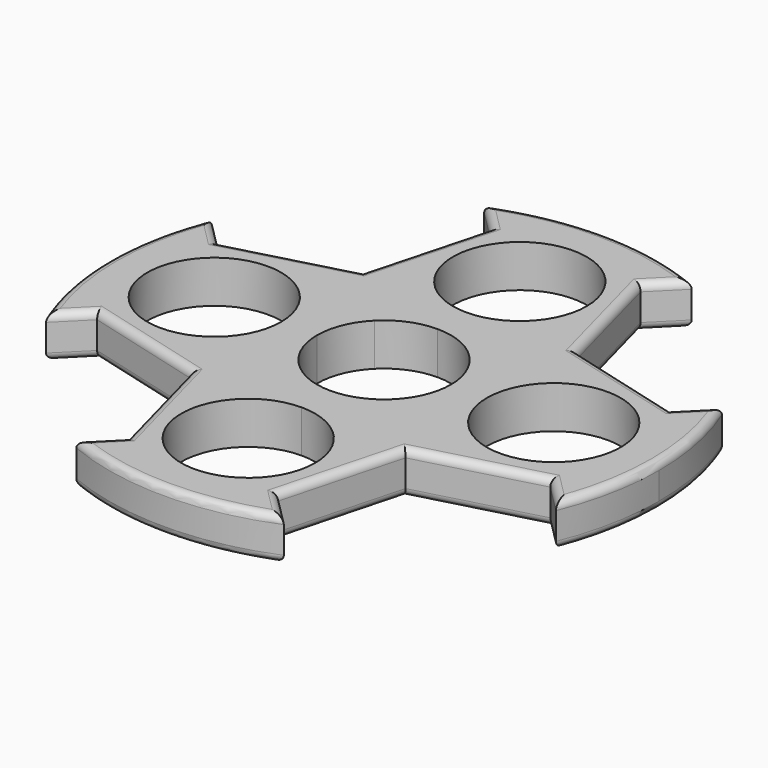
from build123d import *

# Parameters (mm, degrees)
F0_R          = 11.0109
F1_DEPTH      = 6.985
F2_T4_DEPTH   = 26.67
F2_T10_DEPTH  = 12.952299935
F2_T13_ANGLE  = 52.3145955419
F2_T17_DEPTH  = 12.952299935
F2_T22_DEPTH  = 26.67
F2_T28_DEPTH  = 26.67
F2_T34_DEPTH  = 26.67
F2_T40_DEPTH  = 12.952299935
F2_T45_DEPTH  = 12.952299935
F2_T50_DEPTH  = 26.67
F2_T54_ANGLE  = 52.3145955419
F2_T58_DEPTH  = 26.67
F2_T64_DEPTH  = 12.952299935
F2_T67_ANGLE  = 52.3145955419
F2_T71_DEPTH  = 12.952299935
F2_T76_DEPTH  = 26.67
F2_T82_DEPTH  = 26.67
F2_T88_DEPTH  = 12.952299935
F2_T93_DEPTH  = 12.952299935
F2_T96_ANGLE  = 52.3145955419
F2_T98_ANGLE  = 52.3145955419
F2_T102_DEPTH = 26.67
F2_T108_DEPTH = 26.67
F2_T114_DEPTH = 12.952299935
F2_T117_ANGLE = 52.3145955419
F2_T121_DEPTH = 26.67
F2_T127_DEPTH = 12.952299935
F2_T132_DEPTH = 26.67
F2_T138_DEPTH = 12.952299935
F2_T141_ANGLE = 52.3145955419
F2_T145_DEPTH = 12.952299935
F2_T150_DEPTH = 26.67
F2_T156_DEPTH = 26.67
F2_T162_DEPTH = 12.952299935
F2_T165_ANGLE = 52.3145955419
F2_T169_DEPTH = 26.67
F2_T175_DEPTH = 12.952299935
F2_T180_DEPTH = 26.67
F2_T186_DEPTH = 12.952299935
F2_T192_DEPTH = 12.952299935
F2_T196_DEPTH = 26.67
F2_T203_DEPTH = 26.67
F2_T207_DEPTH = 26.67
F2_T214_DEPTH = 26.67
F2_T218_DEPTH = 12.952299935
F2_T225_DEPTH = 26.67
F2_T229_DEPTH = 26.67
F2_T236_DEPTH = 12.952299935
F2_T240_DEPTH = 26.67
F2_T247_DEPTH = 26.67
F2_T251_DEPTH = 12.952299935
F2_T258_DEPTH = 12.952299935
F2_T262_DEPTH = 26.67
F2_T269_DEPTH = 26.67
F2_T273_DEPTH = 26.67
F2_T280_DEPTH = 26.67
F2_T284_DEPTH = 12.952299935
F2_T291_DEPTH = 12.952299935
F2_T295_DEPTH = 26.67
F2_T302_DEPTH = 26.67
F2_T306_DEPTH = 26.67
F2_T313_DEPTH = 26.67
F2_T317_DEPTH = 12.952299935
F2_T324_DEPTH = 26.67
F2_T328_DEPTH = 26.67
F2_T335_DEPTH = 26.67
F2_T339_DEPTH = 12.952299935
F2_T346_DEPTH = 12.952299935
F2_T350_DEPTH = 26.67
F2_T357_DEPTH = 26.67
F2_T361_DEPTH = 26.67
F2_T368_DEPTH = 26.67
F2_T372_DEPTH = 12.952299935
F2_T379_DEPTH = 12.952299935
F2_T383_DEPTH = 26.67
F2_T390_DEPTH = 26.67
F2_T394_DEPTH = 26.67
F2_T401_DEPTH = 26.67
F2_T405_DEPTH = 12.952299935
F2_T412_DEPTH = 12.952299935
F2_T416_DEPTH = 26.67
F2_T423_DEPTH = 26.67
F2_T427_DEPTH = 26.67
F2_T434_DEPTH = 26.67
F2_T438_DEPTH = 12.952299935


# Not quite as in the source:
# - a fillet or chamfer that OpenCascade refuses, or shapes differently, is made with other operations: its cross-section is extruded or revolved along the edge and cut away or added


with BuildPart() as f1:
    # F0 (on Top) → F1 (new body)
    with BuildSketch(Plane.XY):
        with BuildLine():
            ThreePointArc((7.785882057, 7.785882057), (10.1727451445, 4.2136890054), (11.0109, 0))
            ThreePointArc((11.0109, 0), (10.1727451445, -4.2136890054), (7.785882057, -7.785882057))
            Line((7.785882057, -7.785882057), (17.6641637901, -17.6641637901))
            Line((17.6641637901, -17.6641637901), (37.2917765803, -12.4049607937))
            Line((37.2917765803, -12.4049607937), (41.9603076358, -17.0734918491))
            ThreePointArc((41.9603076358, -17.0734918491), (44.4579084134, -8.698616), (45.3009, 0))
            ThreePointArc((45.3009, 0), (44.4579084134, 8.698616), (41.9603076358, 17.0734918491))
            Line((41.9603076358, 17.0734918491), (37.2917765803, 12.4049607937))
            Line((37.2917765803, 12.4049607937), (17.6641637901, 17.6641637901))
            Line((17.6641637901, 17.6641637901), (7.785882057, 7.785882057))
        make_face()
        with BuildLine():
            ThreePointArc((38.9509, 0), (27.94, -11.0109), (16.9291, 0))
            ThreePointArc((16.9291, 0), (27.94, 11.0109), (38.9509, 0))
        make_face(mode=Mode.SUBTRACT)
        with BuildLine():
            ThreePointArc((0, 11.0109), (4.2136890054, 10.1727451445), (7.785882057, 7.785882057))
            Line((7.785882057, 7.785882057), (17.6641637901, 17.6641637901))
            Line((17.6641637901, 17.6641637901), (12.4049607937, 37.2917765803))
            Line((12.4049607937, 37.2917765803), (17.0734918491, 41.9603076358))
            ThreePointArc((17.0734918491, 41.9603076358), (0, 45.3009), (-17.0734918491, 41.9603076358))
            Line((-17.0734918491, 41.9603076358), (-12.4049607937, 37.2917765803))
            Line((-12.4049607937, 37.2917765803), (-17.6641637901, 17.6641637901))
            Line((-17.6641637901, 17.6641637901), (-7.785882057, 7.785882057))
            ThreePointArc((-7.785882057, 7.785882057), (-4.2136890054, 10.1727451445), (0, 11.0109))
        make_face()
        with BuildLine():
            ThreePointArc((11.0109, 27.94), (7.785882057, 20.154117943), (0, 16.9291))
            ThreePointArc((0, 16.9291), (-7.785882057, 35.725882057), (11.0109, 27.94))
        make_face(mode=Mode.SUBTRACT)
        with BuildLine():
            ThreePointArc((-7.785882057, -7.785882057), (-10.1727451445, -4.2136890054), (-11.0109, 0))
            ThreePointArc((-11.0109, 0), (-10.1727451445, 4.2136890054), (-7.785882057, 7.785882057))
            Line((-7.785882057, 7.785882057), (-17.6641637901, 17.6641637901))
            Line((-17.6641637901, 17.6641637901), (-37.2917765803, 12.4049607937))
            Line((-37.2917765803, 12.4049607937), (-41.9603076358, 17.0734918491))
            ThreePointArc((-41.9603076358, 17.0734918491), (-45.3009, 0), (-41.9603076358, -17.0734918491))
            Line((-41.9603076358, -17.0734918491), (-37.2917765803, -12.4049607937))
            Line((-37.2917765803, -12.4049607937), (-17.6641637901, -17.6641637901))
            Line((-17.6641637901, -17.6641637901), (-7.785882057, -7.785882057))
        make_face()
        with Locations((-27.94, 0)):
            Circle(F0_R, mode=Mode.SUBTRACT)
        with BuildLine():
            Line((17.6641637901, -17.6641637901), (7.785882057, -7.785882057))
            ThreePointArc((7.785882057, -7.785882057), (4.2136890054, -10.1727451445), (0, -11.0109))
            ThreePointArc((0, -11.0109), (-4.2136890054, -10.1727451445), (-7.785882057, -7.785882057))
            Line((-7.785882057, -7.785882057), (-17.6641637901, -17.6641637901))
            Line((-17.6641637901, -17.6641637901), (-12.4049607937, -37.2917765803))
            Line((-12.4049607937, -37.2917765803), (-17.0734918491, -41.9603076358))
            ThreePointArc((-17.0734918491, -41.9603076358), (0, -45.3009), (17.0734918491, -41.9603076358))
            Line((17.0734918491, -41.9603076358), (12.4049607937, -37.2917765803))
            Line((12.4049607937, -37.2917765803), (17.6641637901, -17.6641637901))
        make_face()
        with BuildLine():
            ThreePointArc((11.0109, -27.94), (-7.785882057, -35.725882057), (0, -16.9291))
            ThreePointArc((0, -16.9291), (7.785882057, -20.154117943), (11.0109, -27.94))
        make_face(mode=Mode.SUBTRACT)
    extrude(amount=F1_DEPTH)

    # F2: fillet of radius 1.27 on 39 edges, made by hand


with BuildPart() as f2_tool2:
    # F2_s3 → F2_t4 (new body)
    with BuildSketch(Plane(origin=(9.3137198066, 34.7592755256, 0), x_dir=(0, 0, 1), z_dir=(-0.2588190451, -0.9659258263, 0))):
        with BuildLine():
            ThreePointArc((5.715, 21.6340940094), (6.6130256121, 21.2621196215), (6.985, 20.3640940094))
            Line((6.985, 20.3640940094), (6.985, 21.6340940094))
            Line((6.985, 21.6340940094), (5.715, 21.6340940094))
        make_face()
    extrude(amount=F2_T4_DEPTH)

    split(bisect_by=Plane(origin=(12.4434078933, 12.4434078933, 0), x_dir=(0, 0, 1), z_dir=(-0.7071067812, -0.7071067812, 0)), keep=Keep.TOP)

    split(bisect_by=Plane(origin=(-5.5993155532, 20.896930132, 0), x_dir=(0, 0, 1), z_dir=(-0.2588190451, 0.9659258263, 0)), keep=Keep.TOP)


with BuildPart() as f1_1:
    add(f1.part)

    # F2_t1: cut F2_tool2
    add(f2_tool2.part, mode=Mode.SUBTRACT)


with BuildPart() as f2_tool8:
    # F2_s9 → F2_t10 (new body)
    with BuildSketch(Plane(origin=(-31.7619637727, 31.7619637727, 0), x_dir=(0, 0, 1), z_dir=(0.7071067812, -0.7071067812, 0))):
        with BuildLine():
            ThreePointArc((5.715, -17.5976362049), (6.6130256121, -17.9696105928), (6.985, -18.8676362049))
            Line((6.985, -18.8676362049), (6.985, -17.5976362049))
            Line((6.985, -17.5976362049), (5.715, -17.5976362049))
        make_face()
    extrude(amount=F2_T10_DEPTH)

    split(bisect_by=Plane(origin=(-20.896930132, 5.5993155532, 0), x_dir=(0, 0, 1), z_dir=(-0.9659258263, 0.2588190451, 0)), keep=Keep.TOP)


with BuildPart() as f1_2:
    add(f1_1.part)

    # F2_t7: cut F2_tool8
    add(f2_tool8.part, mode=Mode.SUBTRACT)

    # F2_s12 → F2_t13 (revolve, cut)
    with BuildSketch(Plane(origin=(0, 0, 0), x_dir=(0, 0, 1), z_dir=(0.8975871723, -0.4408370085, 0))):
        with BuildLine():
            ThreePointArc((5.715, -45.3009), (6.6130256121, -44.9289256121), (6.985, -44.0309))
            Line((6.985, -44.0309), (6.985, -45.3009))
            Line((6.985, -45.3009), (5.715, -45.3009))
        make_face()
    revolve(axis=Axis((0, 0, 6.985), (0, 0, 1)), revolution_arc=F2_T13_ANGLE, mode=Mode.SUBTRACT)


with BuildPart() as f2_tool15:
    # F2_s16 → F2_t17 (new body)
    with BuildSketch(Plane(origin=(22.6033046567, 22.6033046567, 0), x_dir=(0, 0, 1), z_dir=(0.7071067812, 0.7071067812, 0))):
        with BuildLine():
            ThreePointArc((5.715, -17.5976362049), (6.6130256121, -17.9696105928), (6.985, -18.8676362049))
            Line((6.985, -18.8676362049), (6.985, -17.5976362049))
            Line((6.985, -17.5976362049), (5.715, -17.5976362049))
        make_face()
    extrude(amount=F2_T17_DEPTH)

    split(bisect_by=Plane(origin=(20.896930132, 5.5993155532, 0), x_dir=(0, 0, 1), z_dir=(0.9659258263, 0.2588190451, 0)), keep=Keep.TOP)


with BuildPart() as f1_3:
    add(f1_2.part)

    # F2_t14: cut F2_tool15
    add(f2_tool15.part, mode=Mode.SUBTRACT)


with BuildPart() as f2_tool20:
    # F2_s21 → F2_t22 (new body)
    with BuildSketch(Plane(origin=(-2.4110158737, 8.9980337385, 0), x_dir=(0, 0, 1), z_dir=(-0.2588190451, 0.9659258263, 0))):
        with BuildLine():
            ThreePointArc((5.715, 21.6340940094), (6.6130256121, 21.2621196215), (6.985, 20.3640940094))
            Line((6.985, 20.3640940094), (6.985, 21.6340940094))
            Line((6.985, 21.6340940094), (5.715, 21.6340940094))
        make_face()
    extrude(amount=F2_T22_DEPTH)

    split(bisect_by=Plane(origin=(5.5993155532, 20.896930132, 0), x_dir=(0, 0, 1), z_dir=(0.2588190451, 0.9659258263, 0)), keep=Keep.TOP)

    split(bisect_by=Plane(origin=(-12.4434078933, 12.4434078933, 0), x_dir=(0, 0, 1), z_dir=(0.7071067812, -0.7071067812, 0)), keep=Keep.TOP)


with BuildPart() as f1_4:
    add(f1_3.part)

    # F2_t19: cut F2_tool20
    add(f2_tool20.part, mode=Mode.SUBTRACT)


with BuildPart() as f2_tool26:
    # F2_s27 → F2_t28 (new body)
    with BuildSketch(Plane(origin=(34.7592755256, -9.3137198066, 0), x_dir=(0, 0, 1), z_dir=(-0.9659258263, 0.2588190451, 0))):
        with BuildLine():
            ThreePointArc((5.715, 21.6340940094), (6.6130256121, 21.2621196215), (6.985, 20.3640940094))
            Line((6.985, 20.3640940094), (6.985, 21.6340940094))
            Line((6.985, 21.6340940094), (5.715, 21.6340940094))
        make_face()
    extrude(amount=F2_T28_DEPTH)

    split(bisect_by=Plane(origin=(12.4434078933, -12.4434078933, 0), x_dir=(0, 0, 1), z_dir=(-0.7071067812, 0.7071067812, 0)), keep=Keep.TOP)

    split(bisect_by=Plane(origin=(20.896930132, 5.5993155532, 0), x_dir=(0, 0, 1), z_dir=(0.9659258263, 0.2588190451, 0)), keep=Keep.TOP)


with BuildPart() as f1_5:
    add(f1_4.part)

    # F2_t25: cut F2_tool26
    add(f2_tool26.part, mode=Mode.SUBTRACT)


with BuildPart() as f2_tool32:
    # F2_s33 → F2_t34 (new body)
    with BuildSketch(Plane(origin=(-8.9980337385, -2.4110158737, 0), x_dir=(0, 0, 1), z_dir=(-0.9659258263, -0.2588190451, 0))):
        with BuildLine():
            ThreePointArc((5.715, 21.6340940094), (6.6130256121, 21.2621196215), (6.985, 20.3640940094))
            Line((6.985, 20.3640940094), (6.985, 21.6340940094))
            Line((6.985, 21.6340940094), (5.715, 21.6340940094))
        make_face()
    extrude(amount=F2_T34_DEPTH)

    split(bisect_by=Plane(origin=(-20.896930132, 5.5993155532, 0), x_dir=(0, 0, 1), z_dir=(-0.9659258263, 0.2588190451, 0)), keep=Keep.TOP)

    split(bisect_by=Plane(origin=(-12.4434078933, -12.4434078933, 0), x_dir=(0, 0, 1), z_dir=(0.7071067812, 0.7071067812, 0)), keep=Keep.TOP)


with BuildPart() as f1_6:
    add(f1_5.part)

    # F2_t31: cut F2_tool32
    add(f2_tool32.part, mode=Mode.SUBTRACT)


with BuildPart() as f2_tool38:
    # F2_s39 → F2_t40 (new body)
    with BuildSketch(Plane(origin=(-22.6033046567, 22.6033046567, 0), x_dir=(0, 0, 1), z_dir=(-0.7071067812, 0.7071067812, 0))):
        with BuildLine():
            ThreePointArc((5.715, -17.5976362049), (6.6130256121, -17.9696105928), (6.985, -18.8676362049))
            Line((6.985, -18.8676362049), (6.985, -17.5976362049))
            Line((6.985, -17.5976362049), (5.715, -17.5976362049))
        make_face()
    extrude(amount=F2_T40_DEPTH)

    split(bisect_by=Plane(origin=(-5.5993155532, 20.896930132, 0), x_dir=(0, 0, 1), z_dir=(-0.2588190451, 0.9659258263, 0)), keep=Keep.TOP)


with BuildPart() as f1_7:
    add(f1_6.part)

    # F2_t37: cut F2_tool38
    add(f2_tool38.part, mode=Mode.SUBTRACT)


with BuildPart() as f2_tool43:
    # F2_s44 → F2_t45 (new body)
    with BuildSketch(Plane(origin=(-31.7619637727, -31.7619637727, 0), x_dir=(0, 0, 1), z_dir=(0.7071067812, 0.7071067812, 0))):
        with BuildLine():
            ThreePointArc((5.715, -17.5976362049), (6.6130256121, -17.9696105928), (6.985, -18.8676362049))
            Line((6.985, -18.8676362049), (6.985, -17.5976362049))
            Line((6.985, -17.5976362049), (5.715, -17.5976362049))
        make_face()
    extrude(amount=F2_T45_DEPTH)

    split(bisect_by=Plane(origin=(-5.5993155532, -20.896930132, 0), x_dir=(0, 0, 1), z_dir=(-0.2588190451, -0.9659258263, 0)), keep=Keep.TOP)


with BuildPart() as f1_8:
    add(f1_7.part)

    # F2_t42: cut F2_tool43
    add(f2_tool43.part, mode=Mode.SUBTRACT)


with BuildPart() as f2_tool48:
    # F2_s49 → F2_t50 (new body)
    with BuildSketch(Plane(origin=(-34.7592755256, 9.3137198066, 0), x_dir=(0, 0, 1), z_dir=(0.9659258263, -0.2588190451, 0))):
        with BuildLine():
            ThreePointArc((5.715, 21.6340940094), (6.6130256121, 21.2621196215), (6.985, 20.3640940094))
            Line((6.985, 20.3640940094), (6.985, 21.6340940094))
            Line((6.985, 21.6340940094), (5.715, 21.6340940094))
        make_face()
    extrude(amount=F2_T50_DEPTH)

    split(bisect_by=Plane(origin=(-12.4434078933, 12.4434078933, 0), x_dir=(0, 0, 1), z_dir=(0.7071067812, -0.7071067812, 0)), keep=Keep.TOP)

    split(bisect_by=Plane(origin=(-20.896930132, -5.5993155532, 0), x_dir=(0, 0, 1), z_dir=(-0.9659258263, -0.2588190451, 0)), keep=Keep.TOP)


with BuildPart() as f1_9:
    add(f1_8.part)

    # F2_t47: cut F2_tool48
    add(f2_tool48.part, mode=Mode.SUBTRACT)

    # F2_s53 → F2_t54 (revolve, cut)
    with BuildSketch(Plane(origin=(0, 0, 0), x_dir=(0, 0, 1), z_dir=(0.4408370085, 0.8975871723, 0))):
        with BuildLine():
            ThreePointArc((5.715, -45.3009), (6.6130256121, -44.9289256121), (6.985, -44.0309))
            Line((6.985, -44.0309), (6.985, -45.3009))
            Line((6.985, -45.3009), (5.715, -45.3009))
        make_face()
    revolve(axis=Axis((0, 0, 6.985), (0, 0, 1)), revolution_arc=F2_T54_ANGLE, mode=Mode.SUBTRACT)


with BuildPart() as f2_tool56:
    # F2_s57 → F2_t58 (new body)
    with BuildSketch(Plane(origin=(2.4110158737, -8.9980337385, 0), x_dir=(0, 0, 1), z_dir=(0.2588190451, -0.9659258263, 0))):
        with BuildLine():
            ThreePointArc((5.715, 21.6340940094), (6.6130256121, 21.2621196215), (6.985, 20.3640940094))
            Line((6.985, 20.3640940094), (6.985, 21.6340940094))
            Line((6.985, 21.6340940094), (5.715, 21.6340940094))
        make_face()
    extrude(amount=F2_T58_DEPTH)

    split(bisect_by=Plane(origin=(-5.5993155532, -20.896930132, 0), x_dir=(0, 0, 1), z_dir=(-0.2588190451, -0.9659258263, 0)), keep=Keep.TOP)

    split(bisect_by=Plane(origin=(12.4434078933, -12.4434078933, 0), x_dir=(0, 0, 1), z_dir=(-0.7071067812, 0.7071067812, 0)), keep=Keep.TOP)


with BuildPart() as f1_10:
    add(f1_9.part)

    # F2_t55: cut F2_tool56
    add(f2_tool56.part, mode=Mode.SUBTRACT)


with BuildPart() as f2_tool62:
    # F2_s63 → F2_t64 (new body)
    with BuildSketch(Plane(origin=(-22.6033046567, -22.6033046567, 0), x_dir=(0, 0, 1), z_dir=(-0.7071067812, -0.7071067812, 0))):
        with BuildLine():
            ThreePointArc((5.715, -17.5976362049), (6.6130256121, -17.9696105928), (6.985, -18.8676362049))
            Line((6.985, -18.8676362049), (6.985, -17.5976362049))
            Line((6.985, -17.5976362049), (5.715, -17.5976362049))
        make_face()
    extrude(amount=F2_T64_DEPTH)

    split(bisect_by=Plane(origin=(-20.896930132, -5.5993155532, 0), x_dir=(0, 0, 1), z_dir=(-0.9659258263, -0.2588190451, 0)), keep=Keep.TOP)


with BuildPart() as f1_11:
    add(f1_10.part)

    # F2_t61: cut F2_tool62
    add(f2_tool62.part, mode=Mode.SUBTRACT)

    # F2_s66 → F2_t67 (revolve, cut)
    with BuildSketch(Plane(origin=(0, 0, 0), x_dir=(0, 0, 1), z_dir=(-0.8975871723, 0.4408370085, 0))):
        with BuildLine():
            ThreePointArc((5.715, -45.3009), (6.6130256121, -44.9289256121), (6.985, -44.0309))
            Line((6.985, -44.0309), (6.985, -45.3009))
            Line((6.985, -45.3009), (5.715, -45.3009))
        make_face()
    revolve(axis=Axis((0, 0, 6.985), (0, 0, 1)), revolution_arc=F2_T67_ANGLE, mode=Mode.SUBTRACT)


with BuildPart() as f2_tool69:
    # F2_s70 → F2_t71 (new body)
    with BuildSketch(Plane(origin=(31.7619637727, -31.7619637727, 0), x_dir=(0, 0, 1), z_dir=(-0.7071067812, 0.7071067812, 0))):
        with BuildLine():
            ThreePointArc((5.715, -17.5976362049), (6.6130256121, -17.9696105928), (6.985, -18.8676362049))
            Line((6.985, -18.8676362049), (6.985, -17.5976362049))
            Line((6.985, -17.5976362049), (5.715, -17.5976362049))
        make_face()
    extrude(amount=F2_T71_DEPTH)

    split(bisect_by=Plane(origin=(20.896930132, -5.5993155532, 0), x_dir=(0, 0, 1), z_dir=(0.9659258263, -0.2588190451, 0)), keep=Keep.TOP)


with BuildPart() as f1_12:
    add(f1_11.part)

    # F2_t68: cut F2_tool69
    add(f2_tool69.part, mode=Mode.SUBTRACT)


with BuildPart() as f2_tool74:
    # F2_s75 → F2_t76 (new body)
    with BuildSketch(Plane(origin=(-9.3137198066, -34.7592755256, 0), x_dir=(0, 0, 1), z_dir=(0.2588190451, 0.9659258263, 0))):
        with BuildLine():
            ThreePointArc((5.715, 21.6340940094), (6.6130256121, 21.2621196215), (6.985, 20.3640940094))
            Line((6.985, 20.3640940094), (6.985, 21.6340940094))
            Line((6.985, 21.6340940094), (5.715, 21.6340940094))
        make_face()
    extrude(amount=F2_T76_DEPTH)

    split(bisect_by=Plane(origin=(-12.4434078933, -12.4434078933, 0), x_dir=(0, 0, 1), z_dir=(0.7071067812, 0.7071067812, 0)), keep=Keep.TOP)

    split(bisect_by=Plane(origin=(5.5993155532, -20.896930132, 0), x_dir=(0, 0, 1), z_dir=(0.2588190451, -0.9659258263, 0)), keep=Keep.TOP)


with BuildPart() as f1_13:
    add(f1_12.part)

    # F2_t73: cut F2_tool74
    add(f2_tool74.part, mode=Mode.SUBTRACT)


with BuildPart() as f2_tool80:
    # F2_s81 → F2_t82 (new body)
    with BuildSketch(Plane(origin=(8.9980337385, 2.4110158737, 0), x_dir=(0, 0, 1), z_dir=(0.9659258263, 0.2588190451, 0))):
        with BuildLine():
            ThreePointArc((5.715, 21.6340940094), (6.6130256121, 21.2621196215), (6.985, 20.3640940094))
            Line((6.985, 20.3640940094), (6.985, 21.6340940094))
            Line((6.985, 21.6340940094), (5.715, 21.6340940094))
        make_face()
    extrude(amount=F2_T82_DEPTH)

    split(bisect_by=Plane(origin=(20.896930132, -5.5993155532, 0), x_dir=(0, 0, 1), z_dir=(0.9659258263, -0.2588190451, 0)), keep=Keep.TOP)

    split(bisect_by=Plane(origin=(12.4434078933, 12.4434078933, 0), x_dir=(0, 0, 1), z_dir=(-0.7071067812, -0.7071067812, 0)), keep=Keep.TOP)


with BuildPart() as f1_14:
    add(f1_13.part)

    # F2_t79: cut F2_tool80
    add(f2_tool80.part, mode=Mode.SUBTRACT)


with BuildPart() as f2_tool86:
    # F2_s87 → F2_t88 (new body)
    with BuildSketch(Plane(origin=(22.6033046567, -22.6033046567, 0), x_dir=(0, 0, 1), z_dir=(0.7071067812, -0.7071067812, 0))):
        with BuildLine():
            ThreePointArc((5.715, -17.5976362049), (6.6130256121, -17.9696105928), (6.985, -18.8676362049))
            Line((6.985, -18.8676362049), (6.985, -17.5976362049))
            Line((6.985, -17.5976362049), (5.715, -17.5976362049))
        make_face()
    extrude(amount=F2_T88_DEPTH)

    split(bisect_by=Plane(origin=(5.5993155532, -20.896930132, 0), x_dir=(0, 0, 1), z_dir=(0.2588190451, -0.9659258263, 0)), keep=Keep.TOP)


with BuildPart() as f1_15:
    add(f1_14.part)

    # F2_t85: cut F2_tool86
    add(f2_tool86.part, mode=Mode.SUBTRACT)


with BuildPart() as f2_tool91:
    # F2_s92 → F2_t93 (new body)
    with BuildSketch(Plane(origin=(31.7619637727, 31.7619637727, 0), x_dir=(0, 0, 1), z_dir=(-0.7071067812, -0.7071067812, 0))):
        with BuildLine():
            ThreePointArc((5.715, -17.5976362049), (6.6130256121, -17.9696105928), (6.985, -18.8676362049))
            Line((6.985, -18.8676362049), (6.985, -17.5976362049))
            Line((6.985, -17.5976362049), (5.715, -17.5976362049))
        make_face()
    extrude(amount=F2_T93_DEPTH)

    split(bisect_by=Plane(origin=(5.5993155532, 20.896930132, 0), x_dir=(0, 0, 1), z_dir=(0.2588190451, 0.9659258263, 0)), keep=Keep.TOP)


with BuildPart() as f1_16:
    add(f1_15.part)

    # F2_t90: cut F2_tool91
    add(f2_tool91.part, mode=Mode.SUBTRACT)

    # F2_s95 → F2_t96 (revolve, cut)
    with BuildSketch(Plane(origin=(0, 0, 0), x_dir=(0, 0, 1), z_dir=(-0.4408370085, -0.8975871723, 0))):
        with BuildLine():
            ThreePointArc((5.715, -45.3009), (6.6130256121, -44.9289256121), (6.985, -44.0309))
            Line((6.985, -44.0309), (6.985, -45.3009))
            Line((6.985, -45.3009), (5.715, -45.3009))
        make_face()
    revolve(axis=Axis((0, 0, 6.985), (0, 0, 1)), revolution_arc=F2_T96_ANGLE, mode=Mode.SUBTRACT)

    # F2_s97 → F2_t98 (revolve, cut)
    with BuildSketch(Plane(origin=(0, 0, 0), x_dir=(0, 0, 1), z_dir=(0.8975871723, -0.4408370085, 0))):
        with BuildLine():
            ThreePointArc((1.27, -45.3009), (0.3719743879, -44.9289256121), (0, -44.0309))
            Line((0, -44.0309), (0, -45.3009))
            Line((0, -45.3009), (1.27, -45.3009))
        make_face()
    revolve(axis=Axis((0, 0, 0), (0, 0, 1)), revolution_arc=F2_T98_ANGLE, mode=Mode.SUBTRACT)


with BuildPart() as f2_tool100:
    # F2_s101 → F2_t102 (new body)
    with BuildSketch(Plane(origin=(9.3137198066, 34.7592755256, 0), x_dir=(0, 0, 1), z_dir=(-0.2588190451, -0.9659258263, 0))):
        with BuildLine():
            ThreePointArc((1.27, 21.6340940094), (0.3719743879, 21.2621196215), (0, 20.3640940094))
            Line((0, 20.3640940094), (0, 21.6340940094))
            Line((0, 21.6340940094), (1.27, 21.6340940094))
        make_face()
    extrude(amount=F2_T102_DEPTH)

    split(bisect_by=Plane(origin=(12.4434078933, 12.4434078933, 0), x_dir=(0, 0, 1), z_dir=(-0.7071067812, -0.7071067812, 0)), keep=Keep.TOP)

    split(bisect_by=Plane(origin=(-5.5993155532, 20.896930132, 0), x_dir=(0, 0, 1), z_dir=(-0.2588190451, 0.9659258263, 0)), keep=Keep.TOP)


with BuildPart() as f1_17:
    add(f1_16.part)

    # F2_t99: cut F2_tool100
    add(f2_tool100.part, mode=Mode.SUBTRACT)


with BuildPart() as f2_tool106:
    # F2_s107 → F2_t108 (new body)
    with BuildSketch(Plane(origin=(-8.9980337385, -2.4110158737, 0), x_dir=(0, 0, 1), z_dir=(-0.9659258263, -0.2588190451, 0))):
        with BuildLine():
            ThreePointArc((1.27, 21.6340940094), (0.3719743879, 21.2621196215), (0, 20.3640940094))
            Line((0, 20.3640940094), (0, 21.6340940094))
            Line((0, 21.6340940094), (1.27, 21.6340940094))
        make_face()
    extrude(amount=F2_T108_DEPTH)

    split(bisect_by=Plane(origin=(-20.896930132, 5.5993155532, 0), x_dir=(0, 0, 1), z_dir=(-0.9659258263, 0.2588190451, 0)), keep=Keep.TOP)

    split(bisect_by=Plane(origin=(-12.4434078933, -12.4434078933, 0), x_dir=(0, 0, 1), z_dir=(0.7071067812, 0.7071067812, 0)), keep=Keep.TOP)


with BuildPart() as f1_18:
    add(f1_17.part)

    # F2_t105: cut F2_tool106
    add(f2_tool106.part, mode=Mode.SUBTRACT)


with BuildPart() as f2_tool112:
    # F2_s113 → F2_t114 (new body)
    with BuildSketch(Plane(origin=(-22.6033046567, 22.6033046567, 0), x_dir=(0, 0, 1), z_dir=(-0.7071067812, 0.7071067812, 0))):
        with BuildLine():
            ThreePointArc((1.27, -17.5976362049), (0.3719743879, -17.9696105928), (0, -18.8676362049))
            Line((0, -18.8676362049), (0, -17.5976362049))
            Line((0, -17.5976362049), (1.27, -17.5976362049))
        make_face()
    extrude(amount=F2_T114_DEPTH)

    split(bisect_by=Plane(origin=(-5.5993155532, 20.896930132, 0), x_dir=(0, 0, 1), z_dir=(-0.2588190451, 0.9659258263, 0)), keep=Keep.TOP)


with BuildPart() as f1_19:
    add(f1_18.part)

    # F2_t111: cut F2_tool112
    add(f2_tool112.part, mode=Mode.SUBTRACT)

    # F2_s116 → F2_t117 (revolve, cut)
    with BuildSketch(Plane(origin=(0, 0, 0), x_dir=(0, 0, 1), z_dir=(0.4408370085, 0.8975871723, 0))):
        with BuildLine():
            ThreePointArc((1.27, -45.3009), (0.3719743879, -44.9289256121), (0, -44.0309))
            Line((0, -44.0309), (0, -45.3009))
            Line((0, -45.3009), (1.27, -45.3009))
        make_face()
    revolve(axis=Axis((0, 0, 0), (0, 0, 1)), revolution_arc=F2_T117_ANGLE, mode=Mode.SUBTRACT)


with BuildPart() as f2_tool119:
    # F2_s120 → F2_t121 (new body)
    with BuildSketch(Plane(origin=(-34.7592755256, 9.3137198066, 0), x_dir=(0, 0, 1), z_dir=(0.9659258263, -0.2588190451, 0))):
        with BuildLine():
            ThreePointArc((1.27, 21.6340940094), (0.3719743879, 21.2621196215), (0, 20.3640940094))
            Line((0, 20.3640940094), (0, 21.6340940094))
            Line((0, 21.6340940094), (1.27, 21.6340940094))
        make_face()
    extrude(amount=F2_T121_DEPTH)

    split(bisect_by=Plane(origin=(-12.4434078933, 12.4434078933, 0), x_dir=(0, 0, 1), z_dir=(0.7071067812, -0.7071067812, 0)), keep=Keep.TOP)

    split(bisect_by=Plane(origin=(-20.896930132, -5.5993155532, 0), x_dir=(0, 0, 1), z_dir=(-0.9659258263, -0.2588190451, 0)), keep=Keep.TOP)


with BuildPart() as f1_20:
    add(f1_19.part)

    # F2_t118: cut F2_tool119
    add(f2_tool119.part, mode=Mode.SUBTRACT)


with BuildPart() as f2_tool125:
    # F2_s126 → F2_t127 (new body)
    with BuildSketch(Plane(origin=(-31.7619637727, -31.7619637727, 0), x_dir=(0, 0, 1), z_dir=(0.7071067812, 0.7071067812, 0))):
        with BuildLine():
            ThreePointArc((1.27, -17.5976362049), (0.3719743879, -17.9696105928), (0, -18.8676362049))
            Line((0, -18.8676362049), (0, -17.5976362049))
            Line((0, -17.5976362049), (1.27, -17.5976362049))
        make_face()
    extrude(amount=F2_T127_DEPTH)

    split(bisect_by=Plane(origin=(-5.5993155532, -20.896930132, 0), x_dir=(0, 0, 1), z_dir=(-0.2588190451, -0.9659258263, 0)), keep=Keep.TOP)


with BuildPart() as f1_21:
    add(f1_20.part)

    # F2_t124: cut F2_tool125
    add(f2_tool125.part, mode=Mode.SUBTRACT)


with BuildPart() as f2_tool130:
    # F2_s131 → F2_t132 (new body)
    with BuildSketch(Plane(origin=(2.4110158737, -8.9980337385, 0), x_dir=(0, 0, 1), z_dir=(0.2588190451, -0.9659258263, 0))):
        with BuildLine():
            ThreePointArc((1.27, 21.6340940094), (0.3719743879, 21.2621196215), (0, 20.3640940094))
            Line((0, 20.3640940094), (0, 21.6340940094))
            Line((0, 21.6340940094), (1.27, 21.6340940094))
        make_face()
    extrude(amount=F2_T132_DEPTH)

    split(bisect_by=Plane(origin=(-5.5993155532, -20.896930132, 0), x_dir=(0, 0, 1), z_dir=(-0.2588190451, -0.9659258263, 0)), keep=Keep.TOP)

    split(bisect_by=Plane(origin=(12.4434078933, -12.4434078933, 0), x_dir=(0, 0, 1), z_dir=(-0.7071067812, 0.7071067812, 0)), keep=Keep.TOP)


with BuildPart() as f1_22:
    add(f1_21.part)

    # F2_t129: cut F2_tool130
    add(f2_tool130.part, mode=Mode.SUBTRACT)


with BuildPart() as f2_tool136:
    # F2_s137 → F2_t138 (new body)
    with BuildSketch(Plane(origin=(-22.6033046567, -22.6033046567, 0), x_dir=(0, 0, 1), z_dir=(-0.7071067812, -0.7071067812, 0))):
        with BuildLine():
            ThreePointArc((1.27, -17.5976362049), (0.3719743879, -17.9696105928), (0, -18.8676362049))
            Line((0, -18.8676362049), (0, -17.5976362049))
            Line((0, -17.5976362049), (1.27, -17.5976362049))
        make_face()
    extrude(amount=F2_T138_DEPTH)

    split(bisect_by=Plane(origin=(-20.896930132, -5.5993155532, 0), x_dir=(0, 0, 1), z_dir=(-0.9659258263, -0.2588190451, 0)), keep=Keep.TOP)


with BuildPart() as f1_23:
    add(f1_22.part)

    # F2_t135: cut F2_tool136
    add(f2_tool136.part, mode=Mode.SUBTRACT)

    # F2_s140 → F2_t141 (revolve, cut)
    with BuildSketch(Plane(origin=(0, 0, 0), x_dir=(0, 0, 1), z_dir=(-0.8975871723, 0.4408370085, 0))):
        with BuildLine():
            ThreePointArc((1.27, -45.3009), (0.3719743879, -44.9289256121), (0, -44.0309))
            Line((0, -44.0309), (0, -45.3009))
            Line((0, -45.3009), (1.27, -45.3009))
        make_face()
    revolve(axis=Axis((0, 0, 0), (0, 0, 1)), revolution_arc=F2_T141_ANGLE, mode=Mode.SUBTRACT)


with BuildPart() as f2_tool143:
    # F2_s144 → F2_t145 (new body)
    with BuildSketch(Plane(origin=(31.7619637727, -31.7619637727, 0), x_dir=(0, 0, 1), z_dir=(-0.7071067812, 0.7071067812, 0))):
        with BuildLine():
            ThreePointArc((1.27, -17.5976362049), (0.3719743879, -17.9696105928), (0, -18.8676362049))
            Line((0, -18.8676362049), (0, -17.5976362049))
            Line((0, -17.5976362049), (1.27, -17.5976362049))
        make_face()
    extrude(amount=F2_T145_DEPTH)

    split(bisect_by=Plane(origin=(20.896930132, -5.5993155532, 0), x_dir=(0, 0, 1), z_dir=(0.9659258263, -0.2588190451, 0)), keep=Keep.TOP)


with BuildPart() as f1_24:
    add(f1_23.part)

    # F2_t142: cut F2_tool143
    add(f2_tool143.part, mode=Mode.SUBTRACT)


with BuildPart() as f2_tool148:
    # F2_s149 → F2_t150 (new body)
    with BuildSketch(Plane(origin=(-9.3137198066, -34.7592755256, 0), x_dir=(0, 0, 1), z_dir=(0.2588190451, 0.9659258263, 0))):
        with BuildLine():
            ThreePointArc((1.27, 21.6340940094), (0.3719743879, 21.2621196215), (0, 20.3640940094))
            Line((0, 20.3640940094), (0, 21.6340940094))
            Line((0, 21.6340940094), (1.27, 21.6340940094))
        make_face()
    extrude(amount=F2_T150_DEPTH)

    split(bisect_by=Plane(origin=(-12.4434078933, -12.4434078933, 0), x_dir=(0, 0, 1), z_dir=(0.7071067812, 0.7071067812, 0)), keep=Keep.TOP)

    split(bisect_by=Plane(origin=(5.5993155532, -20.896930132, 0), x_dir=(0, 0, 1), z_dir=(0.2588190451, -0.9659258263, 0)), keep=Keep.TOP)


with BuildPart() as f1_25:
    add(f1_24.part)

    # F2_t147: cut F2_tool148
    add(f2_tool148.part, mode=Mode.SUBTRACT)


with BuildPart() as f2_tool154:
    # F2_s155 → F2_t156 (new body)
    with BuildSketch(Plane(origin=(8.9980337385, 2.4110158737, 0), x_dir=(0, 0, 1), z_dir=(0.9659258263, 0.2588190451, 0))):
        with BuildLine():
            ThreePointArc((1.27, 21.6340940094), (0.3719743879, 21.2621196215), (0, 20.3640940094))
            Line((0, 20.3640940094), (0, 21.6340940094))
            Line((0, 21.6340940094), (1.27, 21.6340940094))
        make_face()
    extrude(amount=F2_T156_DEPTH)

    split(bisect_by=Plane(origin=(20.896930132, -5.5993155532, 0), x_dir=(0, 0, 1), z_dir=(0.9659258263, -0.2588190451, 0)), keep=Keep.TOP)

    split(bisect_by=Plane(origin=(12.4434078933, 12.4434078933, 0), x_dir=(0, 0, 1), z_dir=(-0.7071067812, -0.7071067812, 0)), keep=Keep.TOP)


with BuildPart() as f1_26:
    add(f1_25.part)

    # F2_t153: cut F2_tool154
    add(f2_tool154.part, mode=Mode.SUBTRACT)


with BuildPart() as f2_tool160:
    # F2_s161 → F2_t162 (new body)
    with BuildSketch(Plane(origin=(22.6033046567, -22.6033046567, 0), x_dir=(0, 0, 1), z_dir=(0.7071067812, -0.7071067812, 0))):
        with BuildLine():
            ThreePointArc((1.27, -17.5976362049), (0.3719743879, -17.9696105928), (0, -18.8676362049))
            Line((0, -18.8676362049), (0, -17.5976362049))
            Line((0, -17.5976362049), (1.27, -17.5976362049))
        make_face()
    extrude(amount=F2_T162_DEPTH)

    split(bisect_by=Plane(origin=(5.5993155532, -20.896930132, 0), x_dir=(0, 0, 1), z_dir=(0.2588190451, -0.9659258263, 0)), keep=Keep.TOP)


with BuildPart() as f1_27:
    add(f1_26.part)

    # F2_t159: cut F2_tool160
    add(f2_tool160.part, mode=Mode.SUBTRACT)

    # F2_s164 → F2_t165 (revolve, cut)
    with BuildSketch(Plane(origin=(0, 0, 0), x_dir=(0, 0, 1), z_dir=(-0.4408370085, -0.8975871723, 0))):
        with BuildLine():
            ThreePointArc((1.27, -45.3009), (0.3719743879, -44.9289256121), (0, -44.0309))
            Line((0, -44.0309), (0, -45.3009))
            Line((0, -45.3009), (1.27, -45.3009))
        make_face()
    revolve(axis=Axis((0, 0, 0), (0, 0, 1)), revolution_arc=F2_T165_ANGLE, mode=Mode.SUBTRACT)


with BuildPart() as f2_tool167:
    # F2_s168 → F2_t169 (new body)
    with BuildSketch(Plane(origin=(34.7592755256, -9.3137198066, 0), x_dir=(0, 0, 1), z_dir=(-0.9659258263, 0.2588190451, 0))):
        with BuildLine():
            ThreePointArc((1.27, 21.6340940094), (0.3719743879, 21.2621196215), (0, 20.3640940094))
            Line((0, 20.3640940094), (0, 21.6340940094))
            Line((0, 21.6340940094), (1.27, 21.6340940094))
        make_face()
    extrude(amount=F2_T169_DEPTH)

    split(bisect_by=Plane(origin=(12.4434078933, -12.4434078933, 0), x_dir=(0, 0, 1), z_dir=(-0.7071067812, 0.7071067812, 0)), keep=Keep.TOP)

    split(bisect_by=Plane(origin=(20.896930132, 5.5993155532, 0), x_dir=(0, 0, 1), z_dir=(0.9659258263, 0.2588190451, 0)), keep=Keep.TOP)


with BuildPart() as f1_28:
    add(f1_27.part)

    # F2_t166: cut F2_tool167
    add(f2_tool167.part, mode=Mode.SUBTRACT)


with BuildPart() as f2_tool173:
    # F2_s174 → F2_t175 (new body)
    with BuildSketch(Plane(origin=(31.7619637727, 31.7619637727, 0), x_dir=(0, 0, 1), z_dir=(-0.7071067812, -0.7071067812, 0))):
        with BuildLine():
            ThreePointArc((1.27, -17.5976362049), (0.3719743879, -17.9696105928), (0, -18.8676362049))
            Line((0, -18.8676362049), (0, -17.5976362049))
            Line((0, -17.5976362049), (1.27, -17.5976362049))
        make_face()
    extrude(amount=F2_T175_DEPTH)

    split(bisect_by=Plane(origin=(5.5993155532, 20.896930132, 0), x_dir=(0, 0, 1), z_dir=(0.2588190451, 0.9659258263, 0)), keep=Keep.TOP)


with BuildPart() as f1_29:
    add(f1_28.part)

    # F2_t172: cut F2_tool173
    add(f2_tool173.part, mode=Mode.SUBTRACT)


with BuildPart() as f2_tool178:
    # F2_s179 → F2_t180 (new body)
    with BuildSketch(Plane(origin=(-2.4110158737, 8.9980337385, 0), x_dir=(0, 0, 1), z_dir=(-0.2588190451, 0.9659258263, 0))):
        with BuildLine():
            ThreePointArc((1.27, 21.6340940094), (0.3719743879, 21.2621196215), (0, 20.3640940094))
            Line((0, 20.3640940094), (0, 21.6340940094))
            Line((0, 21.6340940094), (1.27, 21.6340940094))
        make_face()
    extrude(amount=F2_T180_DEPTH)

    split(bisect_by=Plane(origin=(5.5993155532, 20.896930132, 0), x_dir=(0, 0, 1), z_dir=(0.2588190451, 0.9659258263, 0)), keep=Keep.TOP)

    split(bisect_by=Plane(origin=(-12.4434078933, 12.4434078933, 0), x_dir=(0, 0, 1), z_dir=(0.7071067812, -0.7071067812, 0)), keep=Keep.TOP)


with BuildPart() as f1_30:
    add(f1_29.part)

    # F2_t177: cut F2_tool178
    add(f2_tool178.part, mode=Mode.SUBTRACT)


with BuildPart() as f2_tool184:
    # F2_s185 → F2_t186 (new body)
    with BuildSketch(Plane(origin=(22.6033046567, 22.6033046567, 0), x_dir=(0, 0, 1), z_dir=(0.7071067812, 0.7071067812, 0))):
        with BuildLine():
            ThreePointArc((1.27, -17.5976362049), (0.3719743879, -17.9696105928), (0, -18.8676362049))
            Line((0, -18.8676362049), (0, -17.5976362049))
            Line((0, -17.5976362049), (1.27, -17.5976362049))
        make_face()
    extrude(amount=F2_T186_DEPTH)

    split(bisect_by=Plane(origin=(20.896930132, 5.5993155532, 0), x_dir=(0, 0, 1), z_dir=(0.9659258263, 0.2588190451, 0)), keep=Keep.TOP)


with BuildPart() as f1_31:
    add(f1_30.part)

    # F2_t183: cut F2_tool184
    add(f2_tool184.part, mode=Mode.SUBTRACT)


with BuildPart() as f2_tool190:
    # F2_s191 → F2_t192 (new body)
    with BuildSketch(Plane(origin=(-31.7619637727, 31.7619637727, 0), x_dir=(0, 0, 1), z_dir=(0.7071067812, -0.7071067812, 0))):
        with BuildLine():
            ThreePointArc((5.715, -17.5976362049), (6.6130256121, -17.9696105928), (6.985, -18.8676362049))
            Line((6.985, -18.8676362049), (6.985, -17.5976362049))
            Line((6.985, -17.5976362049), (5.715, -17.5976362049))
        make_face()
    extrude(amount=F2_T192_DEPTH)

    split(bisect_by=Plane(origin=(-20.896930132, 5.5993155532, 0), x_dir=(0, 0, 1), z_dir=(0.9659258263, -0.2588190451, 0)), keep=Keep.TOP)


with BuildPart() as f2_tool194:
    # F2_s195 → F2_t196 (new body)
    with BuildSketch(Plane(origin=(9.3137198066, 34.7592755256, 0), x_dir=(0, 0, 1), z_dir=(-0.2588190451, -0.9659258263, 0))):
        with BuildLine():
            ThreePointArc((5.715, 21.6340940094), (6.6130256121, 21.2621196215), (6.985, 20.3640940094))
            Line((6.985, 20.3640940094), (6.985, 21.6340940094))
            Line((6.985, 21.6340940094), (5.715, 21.6340940094))
        make_face()
    extrude(amount=F2_T196_DEPTH)

    split(bisect_by=Plane(origin=(12.4434078933, 12.4434078933, 0), x_dir=(0, 0, 1), z_dir=(0.7071067812, 0.7071067812, 0)), keep=Keep.TOP)


with BuildPart() as f2_tool190_1:
    add(f2_tool190.part)

    # F2_t198: intersect F2_tool194
    add(f2_tool194.part, mode=Mode.INTERSECT)


with BuildPart() as f1_32:
    add(f1_31.part)

    # F2_t188: cut F2_tool190
    add(f2_tool190_1.part, mode=Mode.SUBTRACT)


with BuildPart() as f2_tool201:
    # F2_s202 → F2_t203 (new body)
    with BuildSketch(Plane(origin=(9.3137198066, 34.7592755256, 0), x_dir=(0, 0, 1), z_dir=(-0.2588190451, -0.9659258263, 0))):
        with BuildLine():
            ThreePointArc((5.715, 21.6340940094), (6.6130256121, 21.2621196215), (6.985, 20.3640940094))
            Line((6.985, 20.3640940094), (6.985, 21.6340940094))
            Line((6.985, 21.6340940094), (5.715, 21.6340940094))
        make_face()
    extrude(amount=F2_T203_DEPTH)

    split(bisect_by=Plane(origin=(-5.5993155532, 20.896930132, 0), x_dir=(0, 0, 1), z_dir=(0.2588190451, -0.9659258263, 0)), keep=Keep.TOP)


with BuildPart() as f2_tool205:
    # F2_s206 → F2_t207 (new body)
    with BuildSketch(Plane(origin=(-8.9980337385, -2.4110158737, 0), x_dir=(0, 0, 1), z_dir=(-0.9659258263, -0.2588190451, 0))):
        with BuildLine():
            ThreePointArc((5.715, 21.6340940094), (6.6130256121, 21.2621196215), (6.985, 20.3640940094))
            Line((6.985, 20.3640940094), (6.985, 21.6340940094))
            Line((6.985, 21.6340940094), (5.715, 21.6340940094))
        make_face()
    extrude(amount=F2_T207_DEPTH)

    split(bisect_by=Plane(origin=(-20.896930132, 5.5993155532, 0), x_dir=(0, 0, 1), z_dir=(0.9659258263, -0.2588190451, 0)), keep=Keep.TOP)


with BuildPart() as f2_tool201_1:
    add(f2_tool201.part)

    # F2_t209: intersect F2_tool205
    add(f2_tool205.part, mode=Mode.INTERSECT)


with BuildPart() as f1_33:
    add(f1_32.part)

    # F2_t199: cut F2_tool201
    add(f2_tool201_1.part, mode=Mode.SUBTRACT)


with BuildPart() as f2_tool212:
    # F2_s213 → F2_t214 (new body)
    with BuildSketch(Plane(origin=(-2.4110158737, 8.9980337385, 0), x_dir=(0, 0, 1), z_dir=(-0.2588190451, 0.9659258263, 0))):
        with BuildLine():
            ThreePointArc((5.715, 21.6340940094), (6.6130256121, 21.2621196215), (6.985, 20.3640940094))
            Line((6.985, 20.3640940094), (6.985, 21.6340940094))
            Line((6.985, 21.6340940094), (5.715, 21.6340940094))
        make_face()
    extrude(amount=F2_T214_DEPTH)

    split(bisect_by=Plane(origin=(-12.4434078933, 12.4434078933, 0), x_dir=(0, 0, 1), z_dir=(-0.7071067812, 0.7071067812, 0)), keep=Keep.TOP)


with BuildPart() as f2_tool216:
    # F2_s217 → F2_t218 (new body)
    with BuildSketch(Plane(origin=(22.6033046567, 22.6033046567, 0), x_dir=(0, 0, 1), z_dir=(0.7071067812, 0.7071067812, 0))):
        with BuildLine():
            ThreePointArc((5.715, -17.5976362049), (6.6130256121, -17.9696105928), (6.985, -18.8676362049))
            Line((6.985, -18.8676362049), (6.985, -17.5976362049))
            Line((6.985, -17.5976362049), (5.715, -17.5976362049))
        make_face()
    extrude(amount=F2_T218_DEPTH)

    split(bisect_by=Plane(origin=(20.896930132, 5.5993155532, 0), x_dir=(0, 0, 1), z_dir=(-0.9659258263, -0.2588190451, 0)), keep=Keep.TOP)


with BuildPart() as f2_tool212_1:
    add(f2_tool212.part)

    # F2_t220: intersect F2_tool216
    add(f2_tool216.part, mode=Mode.INTERSECT)


with BuildPart() as f1_34:
    add(f1_33.part)

    # F2_t210: cut F2_tool212
    add(f2_tool212_1.part, mode=Mode.SUBTRACT)


with BuildPart() as f2_tool223:
    # F2_s224 → F2_t225 (new body)
    with BuildSketch(Plane(origin=(34.7592755256, -9.3137198066, 0), x_dir=(0, 0, 1), z_dir=(-0.9659258263, 0.2588190451, 0))):
        with BuildLine():
            ThreePointArc((5.715, 21.6340940094), (6.6130256121, 21.2621196215), (6.985, 20.3640940094))
            Line((6.985, 20.3640940094), (6.985, 21.6340940094))
            Line((6.985, 21.6340940094), (5.715, 21.6340940094))
        make_face()
    extrude(amount=F2_T225_DEPTH)

    split(bisect_by=Plane(origin=(20.896930132, 5.5993155532, 0), x_dir=(0, 0, 1), z_dir=(-0.9659258263, -0.2588190451, 0)), keep=Keep.TOP)


with BuildPart() as f2_tool227:
    # F2_s228 → F2_t229 (new body)
    with BuildSketch(Plane(origin=(-2.4110158737, 8.9980337385, 0), x_dir=(0, 0, 1), z_dir=(-0.2588190451, 0.9659258263, 0))):
        with BuildLine():
            ThreePointArc((5.715, 21.6340940094), (6.6130256121, 21.2621196215), (6.985, 20.3640940094))
            Line((6.985, 20.3640940094), (6.985, 21.6340940094))
            Line((6.985, 21.6340940094), (5.715, 21.6340940094))
        make_face()
    extrude(amount=F2_T229_DEPTH)

    split(bisect_by=Plane(origin=(5.5993155532, 20.896930132, 0), x_dir=(0, 0, 1), z_dir=(-0.2588190451, -0.9659258263, 0)), keep=Keep.TOP)


with BuildPart() as f2_tool223_1:
    add(f2_tool223.part)

    # F2_t231: intersect F2_tool227
    add(f2_tool227.part, mode=Mode.INTERSECT)


with BuildPart() as f1_35:
    add(f1_34.part)

    # F2_t221: cut F2_tool223
    add(f2_tool223_1.part, mode=Mode.SUBTRACT)


with BuildPart() as f2_tool234:
    # F2_s235 → F2_t236 (new body)
    with BuildSketch(Plane(origin=(31.7619637727, 31.7619637727, 0), x_dir=(0, 0, 1), z_dir=(-0.7071067812, -0.7071067812, 0))):
        with BuildLine():
            ThreePointArc((5.715, -17.5976362049), (6.6130256121, -17.9696105928), (6.985, -18.8676362049))
            Line((6.985, -18.8676362049), (6.985, -17.5976362049))
            Line((6.985, -17.5976362049), (5.715, -17.5976362049))
        make_face()
    extrude(amount=F2_T236_DEPTH)

    split(bisect_by=Plane(origin=(5.5993155532, 20.896930132, 0), x_dir=(0, 0, 1), z_dir=(-0.2588190451, -0.9659258263, 0)), keep=Keep.TOP)


with BuildPart() as f2_tool238:
    # F2_s239 → F2_t240 (new body)
    with BuildSketch(Plane(origin=(34.7592755256, -9.3137198066, 0), x_dir=(0, 0, 1), z_dir=(-0.9659258263, 0.2588190451, 0))):
        with BuildLine():
            ThreePointArc((5.715, 21.6340940094), (6.6130256121, 21.2621196215), (6.985, 20.3640940094))
            Line((6.985, 20.3640940094), (6.985, 21.6340940094))
            Line((6.985, 21.6340940094), (5.715, 21.6340940094))
        make_face()
    extrude(amount=F2_T240_DEPTH)

    split(bisect_by=Plane(origin=(12.4434078933, -12.4434078933, 0), x_dir=(0, 0, 1), z_dir=(0.7071067812, -0.7071067812, 0)), keep=Keep.TOP)


with BuildPart() as f2_tool234_1:
    add(f2_tool234.part)

    # F2_t242: intersect F2_tool238
    add(f2_tool238.part, mode=Mode.INTERSECT)


with BuildPart() as f1_36:
    add(f1_35.part)

    # F2_t232: cut F2_tool234
    add(f2_tool234_1.part, mode=Mode.SUBTRACT)


with BuildPart() as f2_tool245:
    # F2_s246 → F2_t247 (new body)
    with BuildSketch(Plane(origin=(-8.9980337385, -2.4110158737, 0), x_dir=(0, 0, 1), z_dir=(-0.9659258263, -0.2588190451, 0))):
        with BuildLine():
            ThreePointArc((5.715, 21.6340940094), (6.6130256121, 21.2621196215), (6.985, 20.3640940094))
            Line((6.985, 20.3640940094), (6.985, 21.6340940094))
            Line((6.985, 21.6340940094), (5.715, 21.6340940094))
        make_face()
    extrude(amount=F2_T247_DEPTH)

    split(bisect_by=Plane(origin=(-12.4434078933, -12.4434078933, 0), x_dir=(0, 0, 1), z_dir=(-0.7071067812, -0.7071067812, 0)), keep=Keep.TOP)


with BuildPart() as f2_tool249:
    # F2_s250 → F2_t251 (new body)
    with BuildSketch(Plane(origin=(-22.6033046567, 22.6033046567, 0), x_dir=(0, 0, 1), z_dir=(-0.7071067812, 0.7071067812, 0))):
        with BuildLine():
            ThreePointArc((5.715, -17.5976362049), (6.6130256121, -17.9696105928), (6.985, -18.8676362049))
            Line((6.985, -18.8676362049), (6.985, -17.5976362049))
            Line((6.985, -17.5976362049), (5.715, -17.5976362049))
        make_face()
    extrude(amount=F2_T251_DEPTH)

    split(bisect_by=Plane(origin=(-5.5993155532, 20.896930132, 0), x_dir=(0, 0, 1), z_dir=(0.2588190451, -0.9659258263, 0)), keep=Keep.TOP)


with BuildPart() as f2_tool245_1:
    add(f2_tool245.part)

    # F2_t253: intersect F2_tool249
    add(f2_tool249.part, mode=Mode.INTERSECT)


with BuildPart() as f1_37:
    add(f1_36.part)

    # F2_t243: cut F2_tool245
    add(f2_tool245_1.part, mode=Mode.SUBTRACT)


with BuildPart() as f2_tool256:
    # F2_s257 → F2_t258 (new body)
    with BuildSketch(Plane(origin=(-31.7619637727, -31.7619637727, 0), x_dir=(0, 0, 1), z_dir=(0.7071067812, 0.7071067812, 0))):
        with BuildLine():
            ThreePointArc((5.715, -17.5976362049), (6.6130256121, -17.9696105928), (6.985, -18.8676362049))
            Line((6.985, -18.8676362049), (6.985, -17.5976362049))
            Line((6.985, -17.5976362049), (5.715, -17.5976362049))
        make_face()
    extrude(amount=F2_T258_DEPTH)

    split(bisect_by=Plane(origin=(-5.5993155532, -20.896930132, 0), x_dir=(0, 0, 1), z_dir=(0.2588190451, 0.9659258263, 0)), keep=Keep.TOP)


with BuildPart() as f2_tool260:
    # F2_s261 → F2_t262 (new body)
    with BuildSketch(Plane(origin=(-34.7592755256, 9.3137198066, 0), x_dir=(0, 0, 1), z_dir=(0.9659258263, -0.2588190451, 0))):
        with BuildLine():
            ThreePointArc((5.715, 21.6340940094), (6.6130256121, 21.2621196215), (6.985, 20.3640940094))
            Line((6.985, 20.3640940094), (6.985, 21.6340940094))
            Line((6.985, 21.6340940094), (5.715, 21.6340940094))
        make_face()
    extrude(amount=F2_T262_DEPTH)

    split(bisect_by=Plane(origin=(-12.4434078933, 12.4434078933, 0), x_dir=(0, 0, 1), z_dir=(-0.7071067812, 0.7071067812, 0)), keep=Keep.TOP)


with BuildPart() as f2_tool256_1:
    add(f2_tool256.part)

    # F2_t264: intersect F2_tool260
    add(f2_tool260.part, mode=Mode.INTERSECT)


with BuildPart() as f1_38:
    add(f1_37.part)

    # F2_t254: cut F2_tool256
    add(f2_tool256_1.part, mode=Mode.SUBTRACT)


with BuildPart() as f2_tool267:
    # F2_s268 → F2_t269 (new body)
    with BuildSketch(Plane(origin=(-34.7592755256, 9.3137198066, 0), x_dir=(0, 0, 1), z_dir=(0.9659258263, -0.2588190451, 0))):
        with BuildLine():
            ThreePointArc((5.715, 21.6340940094), (6.6130256121, 21.2621196215), (6.985, 20.3640940094))
            Line((6.985, 20.3640940094), (6.985, 21.6340940094))
            Line((6.985, 21.6340940094), (5.715, 21.6340940094))
        make_face()
    extrude(amount=F2_T269_DEPTH)

    split(bisect_by=Plane(origin=(-20.896930132, -5.5993155532, 0), x_dir=(0, 0, 1), z_dir=(0.9659258263, 0.2588190451, 0)), keep=Keep.TOP)


with BuildPart() as f2_tool271:
    # F2_s272 → F2_t273 (new body)
    with BuildSketch(Plane(origin=(2.4110158737, -8.9980337385, 0), x_dir=(0, 0, 1), z_dir=(0.2588190451, -0.9659258263, 0))):
        with BuildLine():
            ThreePointArc((5.715, 21.6340940094), (6.6130256121, 21.2621196215), (6.985, 20.3640940094))
            Line((6.985, 20.3640940094), (6.985, 21.6340940094))
            Line((6.985, 21.6340940094), (5.715, 21.6340940094))
        make_face()
    extrude(amount=F2_T273_DEPTH)

    split(bisect_by=Plane(origin=(-5.5993155532, -20.896930132, 0), x_dir=(0, 0, 1), z_dir=(0.2588190451, 0.9659258263, 0)), keep=Keep.TOP)


with BuildPart() as f2_tool267_1:
    add(f2_tool267.part)

    # F2_t275: intersect F2_tool271
    add(f2_tool271.part, mode=Mode.INTERSECT)


with BuildPart() as f1_39:
    add(f1_38.part)

    # F2_t265: cut F2_tool267
    add(f2_tool267_1.part, mode=Mode.SUBTRACT)


with BuildPart() as f2_tool278:
    # F2_s279 → F2_t280 (new body)
    with BuildSketch(Plane(origin=(2.4110158737, -8.9980337385, 0), x_dir=(0, 0, 1), z_dir=(0.2588190451, -0.9659258263, 0))):
        with BuildLine():
            ThreePointArc((5.715, 21.6340940094), (6.6130256121, 21.2621196215), (6.985, 20.3640940094))
            Line((6.985, 20.3640940094), (6.985, 21.6340940094))
            Line((6.985, 21.6340940094), (5.715, 21.6340940094))
        make_face()
    extrude(amount=F2_T280_DEPTH)

    split(bisect_by=Plane(origin=(12.4434078933, -12.4434078933, 0), x_dir=(0, 0, 1), z_dir=(0.7071067812, -0.7071067812, 0)), keep=Keep.TOP)


with BuildPart() as f2_tool282:
    # F2_s283 → F2_t284 (new body)
    with BuildSketch(Plane(origin=(-22.6033046567, -22.6033046567, 0), x_dir=(0, 0, 1), z_dir=(-0.7071067812, -0.7071067812, 0))):
        with BuildLine():
            ThreePointArc((5.715, -17.5976362049), (6.6130256121, -17.9696105928), (6.985, -18.8676362049))
            Line((6.985, -18.8676362049), (6.985, -17.5976362049))
            Line((6.985, -17.5976362049), (5.715, -17.5976362049))
        make_face()
    extrude(amount=F2_T284_DEPTH)

    split(bisect_by=Plane(origin=(-20.896930132, -5.5993155532, 0), x_dir=(0, 0, 1), z_dir=(0.9659258263, 0.2588190451, 0)), keep=Keep.TOP)


with BuildPart() as f2_tool278_1:
    add(f2_tool278.part)

    # F2_t286: intersect F2_tool282
    add(f2_tool282.part, mode=Mode.INTERSECT)


with BuildPart() as f1_40:
    add(f1_39.part)

    # F2_t276: cut F2_tool278
    add(f2_tool278_1.part, mode=Mode.SUBTRACT)


with BuildPart() as f2_tool289:
    # F2_s290 → F2_t291 (new body)
    with BuildSketch(Plane(origin=(31.7619637727, -31.7619637727, 0), x_dir=(0, 0, 1), z_dir=(-0.7071067812, 0.7071067812, 0))):
        with BuildLine():
            ThreePointArc((5.715, -17.5976362049), (6.6130256121, -17.9696105928), (6.985, -18.8676362049))
            Line((6.985, -18.8676362049), (6.985, -17.5976362049))
            Line((6.985, -17.5976362049), (5.715, -17.5976362049))
        make_face()
    extrude(amount=F2_T291_DEPTH)

    split(bisect_by=Plane(origin=(20.896930132, -5.5993155532, 0), x_dir=(0, 0, 1), z_dir=(-0.9659258263, 0.2588190451, 0)), keep=Keep.TOP)


with BuildPart() as f2_tool293:
    # F2_s294 → F2_t295 (new body)
    with BuildSketch(Plane(origin=(-9.3137198066, -34.7592755256, 0), x_dir=(0, 0, 1), z_dir=(0.2588190451, 0.9659258263, 0))):
        with BuildLine():
            ThreePointArc((5.715, 21.6340940094), (6.6130256121, 21.2621196215), (6.985, 20.3640940094))
            Line((6.985, 20.3640940094), (6.985, 21.6340940094))
            Line((6.985, 21.6340940094), (5.715, 21.6340940094))
        make_face()
    extrude(amount=F2_T295_DEPTH)

    split(bisect_by=Plane(origin=(-12.4434078933, -12.4434078933, 0), x_dir=(0, 0, 1), z_dir=(-0.7071067812, -0.7071067812, 0)), keep=Keep.TOP)


with BuildPart() as f2_tool289_1:
    add(f2_tool289.part)

    # F2_t297: intersect F2_tool293
    add(f2_tool293.part, mode=Mode.INTERSECT)


with BuildPart() as f1_41:
    add(f1_40.part)

    # F2_t287: cut F2_tool289
    add(f2_tool289_1.part, mode=Mode.SUBTRACT)


with BuildPart() as f2_tool300:
    # F2_s301 → F2_t302 (new body)
    with BuildSketch(Plane(origin=(-9.3137198066, -34.7592755256, 0), x_dir=(0, 0, 1), z_dir=(0.2588190451, 0.9659258263, 0))):
        with BuildLine():
            ThreePointArc((5.715, 21.6340940094), (6.6130256121, 21.2621196215), (6.985, 20.3640940094))
            Line((6.985, 20.3640940094), (6.985, 21.6340940094))
            Line((6.985, 21.6340940094), (5.715, 21.6340940094))
        make_face()
    extrude(amount=F2_T302_DEPTH)

    split(bisect_by=Plane(origin=(5.5993155532, -20.896930132, 0), x_dir=(0, 0, 1), z_dir=(-0.2588190451, 0.9659258263, 0)), keep=Keep.TOP)


with BuildPart() as f2_tool304:
    # F2_s305 → F2_t306 (new body)
    with BuildSketch(Plane(origin=(8.9980337385, 2.4110158737, 0), x_dir=(0, 0, 1), z_dir=(0.9659258263, 0.2588190451, 0))):
        with BuildLine():
            ThreePointArc((5.715, 21.6340940094), (6.6130256121, 21.2621196215), (6.985, 20.3640940094))
            Line((6.985, 20.3640940094), (6.985, 21.6340940094))
            Line((6.985, 21.6340940094), (5.715, 21.6340940094))
        make_face()
    extrude(amount=F2_T306_DEPTH)

    split(bisect_by=Plane(origin=(20.896930132, -5.5993155532, 0), x_dir=(0, 0, 1), z_dir=(-0.9659258263, 0.2588190451, 0)), keep=Keep.TOP)


with BuildPart() as f2_tool300_1:
    add(f2_tool300.part)

    # F2_t308: intersect F2_tool304
    add(f2_tool304.part, mode=Mode.INTERSECT)


with BuildPart() as f1_42:
    add(f1_41.part)

    # F2_t298: cut F2_tool300
    add(f2_tool300_1.part, mode=Mode.SUBTRACT)


with BuildPart() as f2_tool311:
    # F2_s312 → F2_t313 (new body)
    with BuildSketch(Plane(origin=(8.9980337385, 2.4110158737, 0), x_dir=(0, 0, 1), z_dir=(0.9659258263, 0.2588190451, 0))):
        with BuildLine():
            ThreePointArc((5.715, 21.6340940094), (6.6130256121, 21.2621196215), (6.985, 20.3640940094))
            Line((6.985, 20.3640940094), (6.985, 21.6340940094))
            Line((6.985, 21.6340940094), (5.715, 21.6340940094))
        make_face()
    extrude(amount=F2_T313_DEPTH)

    split(bisect_by=Plane(origin=(12.4434078933, 12.4434078933, 0), x_dir=(0, 0, 1), z_dir=(0.7071067812, 0.7071067812, 0)), keep=Keep.TOP)


with BuildPart() as f2_tool315:
    # F2_s316 → F2_t317 (new body)
    with BuildSketch(Plane(origin=(22.6033046567, -22.6033046567, 0), x_dir=(0, 0, 1), z_dir=(0.7071067812, -0.7071067812, 0))):
        with BuildLine():
            ThreePointArc((5.715, -17.5976362049), (6.6130256121, -17.9696105928), (6.985, -18.8676362049))
            Line((6.985, -18.8676362049), (6.985, -17.5976362049))
            Line((6.985, -17.5976362049), (5.715, -17.5976362049))
        make_face()
    extrude(amount=F2_T317_DEPTH)

    split(bisect_by=Plane(origin=(5.5993155532, -20.896930132, 0), x_dir=(0, 0, 1), z_dir=(-0.2588190451, 0.9659258263, 0)), keep=Keep.TOP)


with BuildPart() as f2_tool311_1:
    add(f2_tool311.part)

    # F2_t319: intersect F2_tool315
    add(f2_tool315.part, mode=Mode.INTERSECT)


with BuildPart() as f1_43:
    add(f1_42.part)

    # F2_t309: cut F2_tool311
    add(f2_tool311_1.part, mode=Mode.SUBTRACT)


with BuildPart() as f2_tool322:
    # F2_s323 → F2_t324 (new body)
    with BuildSketch(Plane(origin=(9.3137198066, 34.7592755256, 0), x_dir=(0, 0, 1), z_dir=(-0.2588190451, -0.9659258263, 0))):
        with BuildLine():
            ThreePointArc((1.27, 21.6340940094), (0.3719743879, 21.2621196215), (0, 20.3640940094))
            Line((0, 20.3640940094), (0, 21.6340940094))
            Line((0, 21.6340940094), (1.27, 21.6340940094))
        make_face()
    extrude(amount=F2_T324_DEPTH)

    split(bisect_by=Plane(origin=(-5.5993155532, 20.896930132, 0), x_dir=(0, 0, 1), z_dir=(0.2588190451, -0.9659258263, 0)), keep=Keep.TOP)


with BuildPart() as f2_tool326:
    # F2_s327 → F2_t328 (new body)
    with BuildSketch(Plane(origin=(-8.9980337385, -2.4110158737, 0), x_dir=(0, 0, 1), z_dir=(-0.9659258263, -0.2588190451, 0))):
        with BuildLine():
            ThreePointArc((1.27, 21.6340940094), (0.3719743879, 21.2621196215), (0, 20.3640940094))
            Line((0, 20.3640940094), (0, 21.6340940094))
            Line((0, 21.6340940094), (1.27, 21.6340940094))
        make_face()
    extrude(amount=F2_T328_DEPTH)

    split(bisect_by=Plane(origin=(-20.896930132, 5.5993155532, 0), x_dir=(0, 0, 1), z_dir=(0.9659258263, -0.2588190451, 0)), keep=Keep.TOP)


with BuildPart() as f2_tool322_1:
    add(f2_tool322.part)

    # F2_t330: intersect F2_tool326
    add(f2_tool326.part, mode=Mode.INTERSECT)


with BuildPart() as f1_44:
    add(f1_43.part)

    # F2_t320: cut F2_tool322
    add(f2_tool322_1.part, mode=Mode.SUBTRACT)


with BuildPart() as f2_tool333:
    # F2_s334 → F2_t335 (new body)
    with BuildSketch(Plane(origin=(-8.9980337385, -2.4110158737, 0), x_dir=(0, 0, 1), z_dir=(-0.9659258263, -0.2588190451, 0))):
        with BuildLine():
            ThreePointArc((1.27, 21.6340940094), (0.3719743879, 21.2621196215), (0, 20.3640940094))
            Line((0, 20.3640940094), (0, 21.6340940094))
            Line((0, 21.6340940094), (1.27, 21.6340940094))
        make_face()
    extrude(amount=F2_T335_DEPTH)

    split(bisect_by=Plane(origin=(-12.4434078933, -12.4434078933, 0), x_dir=(0, 0, 1), z_dir=(-0.7071067812, -0.7071067812, 0)), keep=Keep.TOP)


with BuildPart() as f2_tool337:
    # F2_s338 → F2_t339 (new body)
    with BuildSketch(Plane(origin=(-22.6033046567, 22.6033046567, 0), x_dir=(0, 0, 1), z_dir=(-0.7071067812, 0.7071067812, 0))):
        with BuildLine():
            ThreePointArc((1.27, -17.5976362049), (0.3719743879, -17.9696105928), (0, -18.8676362049))
            Line((0, -18.8676362049), (0, -17.5976362049))
            Line((0, -17.5976362049), (1.27, -17.5976362049))
        make_face()
    extrude(amount=F2_T339_DEPTH)

    split(bisect_by=Plane(origin=(-5.5993155532, 20.896930132, 0), x_dir=(0, 0, 1), z_dir=(0.2588190451, -0.9659258263, 0)), keep=Keep.TOP)


with BuildPart() as f2_tool333_1:
    add(f2_tool333.part)

    # F2_t341: intersect F2_tool337
    add(f2_tool337.part, mode=Mode.INTERSECT)


with BuildPart() as f1_45:
    add(f1_44.part)

    # F2_t331: cut F2_tool333
    add(f2_tool333_1.part, mode=Mode.SUBTRACT)


with BuildPart() as f2_tool344:
    # F2_s345 → F2_t346 (new body)
    with BuildSketch(Plane(origin=(-31.7619637727, -31.7619637727, 0), x_dir=(0, 0, 1), z_dir=(0.7071067812, 0.7071067812, 0))):
        with BuildLine():
            ThreePointArc((1.27, -17.5976362049), (0.3719743879, -17.9696105928), (0, -18.8676362049))
            Line((0, -18.8676362049), (0, -17.5976362049))
            Line((0, -17.5976362049), (1.27, -17.5976362049))
        make_face()
    extrude(amount=F2_T346_DEPTH)

    split(bisect_by=Plane(origin=(-5.5993155532, -20.896930132, 0), x_dir=(0, 0, 1), z_dir=(0.2588190451, 0.9659258263, 0)), keep=Keep.TOP)


with BuildPart() as f2_tool348:
    # F2_s349 → F2_t350 (new body)
    with BuildSketch(Plane(origin=(-34.7592755256, 9.3137198066, 0), x_dir=(0, 0, 1), z_dir=(0.9659258263, -0.2588190451, 0))):
        with BuildLine():
            ThreePointArc((1.27, 21.6340940094), (0.3719743879, 21.2621196215), (0, 20.3640940094))
            Line((0, 20.3640940094), (0, 21.6340940094))
            Line((0, 21.6340940094), (1.27, 21.6340940094))
        make_face()
    extrude(amount=F2_T350_DEPTH)

    split(bisect_by=Plane(origin=(-12.4434078933, 12.4434078933, 0), x_dir=(0, 0, 1), z_dir=(-0.7071067812, 0.7071067812, 0)), keep=Keep.TOP)


with BuildPart() as f2_tool344_1:
    add(f2_tool344.part)

    # F2_t352: intersect F2_tool348
    add(f2_tool348.part, mode=Mode.INTERSECT)


with BuildPart() as f1_46:
    add(f1_45.part)

    # F2_t342: cut F2_tool344
    add(f2_tool344_1.part, mode=Mode.SUBTRACT)


with BuildPart() as f2_tool355:
    # F2_s356 → F2_t357 (new body)
    with BuildSketch(Plane(origin=(-34.7592755256, 9.3137198066, 0), x_dir=(0, 0, 1), z_dir=(0.9659258263, -0.2588190451, 0))):
        with BuildLine():
            ThreePointArc((1.27, 21.6340940094), (0.3719743879, 21.2621196215), (0, 20.3640940094))
            Line((0, 20.3640940094), (0, 21.6340940094))
            Line((0, 21.6340940094), (1.27, 21.6340940094))
        make_face()
    extrude(amount=F2_T357_DEPTH)

    split(bisect_by=Plane(origin=(-20.896930132, -5.5993155532, 0), x_dir=(0, 0, 1), z_dir=(0.9659258263, 0.2588190451, 0)), keep=Keep.TOP)


with BuildPart() as f2_tool359:
    # F2_s360 → F2_t361 (new body)
    with BuildSketch(Plane(origin=(2.4110158737, -8.9980337385, 0), x_dir=(0, 0, 1), z_dir=(0.2588190451, -0.9659258263, 0))):
        with BuildLine():
            ThreePointArc((1.27, 21.6340940094), (0.3719743879, 21.2621196215), (0, 20.3640940094))
            Line((0, 20.3640940094), (0, 21.6340940094))
            Line((0, 21.6340940094), (1.27, 21.6340940094))
        make_face()
    extrude(amount=F2_T361_DEPTH)

    split(bisect_by=Plane(origin=(-5.5993155532, -20.896930132, 0), x_dir=(0, 0, 1), z_dir=(0.2588190451, 0.9659258263, 0)), keep=Keep.TOP)


with BuildPart() as f2_tool355_1:
    add(f2_tool355.part)

    # F2_t363: intersect F2_tool359
    add(f2_tool359.part, mode=Mode.INTERSECT)


with BuildPart() as f1_47:
    add(f1_46.part)

    # F2_t353: cut F2_tool355
    add(f2_tool355_1.part, mode=Mode.SUBTRACT)


with BuildPart() as f2_tool366:
    # F2_s367 → F2_t368 (new body)
    with BuildSketch(Plane(origin=(2.4110158737, -8.9980337385, 0), x_dir=(0, 0, 1), z_dir=(0.2588190451, -0.9659258263, 0))):
        with BuildLine():
            ThreePointArc((1.27, 21.6340940094), (0.3719743879, 21.2621196215), (0, 20.3640940094))
            Line((0, 20.3640940094), (0, 21.6340940094))
            Line((0, 21.6340940094), (1.27, 21.6340940094))
        make_face()
    extrude(amount=F2_T368_DEPTH)

    split(bisect_by=Plane(origin=(12.4434078933, -12.4434078933, 0), x_dir=(0, 0, 1), z_dir=(0.7071067812, -0.7071067812, 0)), keep=Keep.TOP)


with BuildPart() as f2_tool370:
    # F2_s371 → F2_t372 (new body)
    with BuildSketch(Plane(origin=(-22.6033046567, -22.6033046567, 0), x_dir=(0, 0, 1), z_dir=(-0.7071067812, -0.7071067812, 0))):
        with BuildLine():
            ThreePointArc((1.27, -17.5976362049), (0.3719743879, -17.9696105928), (0, -18.8676362049))
            Line((0, -18.8676362049), (0, -17.5976362049))
            Line((0, -17.5976362049), (1.27, -17.5976362049))
        make_face()
    extrude(amount=F2_T372_DEPTH)

    split(bisect_by=Plane(origin=(-20.896930132, -5.5993155532, 0), x_dir=(0, 0, 1), z_dir=(0.9659258263, 0.2588190451, 0)), keep=Keep.TOP)


with BuildPart() as f2_tool366_1:
    add(f2_tool366.part)

    # F2_t374: intersect F2_tool370
    add(f2_tool370.part, mode=Mode.INTERSECT)


with BuildPart() as f1_48:
    add(f1_47.part)

    # F2_t364: cut F2_tool366
    add(f2_tool366_1.part, mode=Mode.SUBTRACT)


with BuildPart() as f2_tool377:
    # F2_s378 → F2_t379 (new body)
    with BuildSketch(Plane(origin=(31.7619637727, -31.7619637727, 0), x_dir=(0, 0, 1), z_dir=(-0.7071067812, 0.7071067812, 0))):
        with BuildLine():
            ThreePointArc((1.27, -17.5976362049), (0.3719743879, -17.9696105928), (0, -18.8676362049))
            Line((0, -18.8676362049), (0, -17.5976362049))
            Line((0, -17.5976362049), (1.27, -17.5976362049))
        make_face()
    extrude(amount=F2_T379_DEPTH)

    split(bisect_by=Plane(origin=(20.896930132, -5.5993155532, 0), x_dir=(0, 0, 1), z_dir=(-0.9659258263, 0.2588190451, 0)), keep=Keep.TOP)


with BuildPart() as f2_tool381:
    # F2_s382 → F2_t383 (new body)
    with BuildSketch(Plane(origin=(-9.3137198066, -34.7592755256, 0), x_dir=(0, 0, 1), z_dir=(0.2588190451, 0.9659258263, 0))):
        with BuildLine():
            ThreePointArc((1.27, 21.6340940094), (0.3719743879, 21.2621196215), (0, 20.3640940094))
            Line((0, 20.3640940094), (0, 21.6340940094))
            Line((0, 21.6340940094), (1.27, 21.6340940094))
        make_face()
    extrude(amount=F2_T383_DEPTH)

    split(bisect_by=Plane(origin=(-12.4434078933, -12.4434078933, 0), x_dir=(0, 0, 1), z_dir=(-0.7071067812, -0.7071067812, 0)), keep=Keep.TOP)


with BuildPart() as f2_tool377_1:
    add(f2_tool377.part)

    # F2_t385: intersect F2_tool381
    add(f2_tool381.part, mode=Mode.INTERSECT)


with BuildPart() as f1_49:
    add(f1_48.part)

    # F2_t375: cut F2_tool377
    add(f2_tool377_1.part, mode=Mode.SUBTRACT)


with BuildPart() as f2_tool388:
    # F2_s389 → F2_t390 (new body)
    with BuildSketch(Plane(origin=(-9.3137198066, -34.7592755256, 0), x_dir=(0, 0, 1), z_dir=(0.2588190451, 0.9659258263, 0))):
        with BuildLine():
            ThreePointArc((1.27, 21.6340940094), (0.3719743879, 21.2621196215), (0, 20.3640940094))
            Line((0, 20.3640940094), (0, 21.6340940094))
            Line((0, 21.6340940094), (1.27, 21.6340940094))
        make_face()
    extrude(amount=F2_T390_DEPTH)

    split(bisect_by=Plane(origin=(5.5993155532, -20.896930132, 0), x_dir=(0, 0, 1), z_dir=(-0.2588190451, 0.9659258263, 0)), keep=Keep.TOP)


with BuildPart() as f2_tool392:
    # F2_s393 → F2_t394 (new body)
    with BuildSketch(Plane(origin=(8.9980337385, 2.4110158737, 0), x_dir=(0, 0, 1), z_dir=(0.9659258263, 0.2588190451, 0))):
        with BuildLine():
            ThreePointArc((1.27, 21.6340940094), (0.3719743879, 21.2621196215), (0, 20.3640940094))
            Line((0, 20.3640940094), (0, 21.6340940094))
            Line((0, 21.6340940094), (1.27, 21.6340940094))
        make_face()
    extrude(amount=F2_T394_DEPTH)

    split(bisect_by=Plane(origin=(20.896930132, -5.5993155532, 0), x_dir=(0, 0, 1), z_dir=(-0.9659258263, 0.2588190451, 0)), keep=Keep.TOP)


with BuildPart() as f2_tool388_1:
    add(f2_tool388.part)

    # F2_t396: intersect F2_tool392
    add(f2_tool392.part, mode=Mode.INTERSECT)


with BuildPart() as f1_50:
    add(f1_49.part)

    # F2_t386: cut F2_tool388
    add(f2_tool388_1.part, mode=Mode.SUBTRACT)


with BuildPart() as f2_tool399:
    # F2_s400 → F2_t401 (new body)
    with BuildSketch(Plane(origin=(8.9980337385, 2.4110158737, 0), x_dir=(0, 0, 1), z_dir=(0.9659258263, 0.2588190451, 0))):
        with BuildLine():
            ThreePointArc((1.27, 21.6340940094), (0.3719743879, 21.2621196215), (0, 20.3640940094))
            Line((0, 20.3640940094), (0, 21.6340940094))
            Line((0, 21.6340940094), (1.27, 21.6340940094))
        make_face()
    extrude(amount=F2_T401_DEPTH)

    split(bisect_by=Plane(origin=(12.4434078933, 12.4434078933, 0), x_dir=(0, 0, 1), z_dir=(0.7071067812, 0.7071067812, 0)), keep=Keep.TOP)


with BuildPart() as f2_tool403:
    # F2_s404 → F2_t405 (new body)
    with BuildSketch(Plane(origin=(22.6033046567, -22.6033046567, 0), x_dir=(0, 0, 1), z_dir=(0.7071067812, -0.7071067812, 0))):
        with BuildLine():
            ThreePointArc((1.27, -17.5976362049), (0.3719743879, -17.9696105928), (0, -18.8676362049))
            Line((0, -18.8676362049), (0, -17.5976362049))
            Line((0, -17.5976362049), (1.27, -17.5976362049))
        make_face()
    extrude(amount=F2_T405_DEPTH)

    split(bisect_by=Plane(origin=(5.5993155532, -20.896930132, 0), x_dir=(0, 0, 1), z_dir=(-0.2588190451, 0.9659258263, 0)), keep=Keep.TOP)


with BuildPart() as f2_tool399_1:
    add(f2_tool399.part)

    # F2_t407: intersect F2_tool403
    add(f2_tool403.part, mode=Mode.INTERSECT)


with BuildPart() as f1_51:
    add(f1_50.part)

    # F2_t397: cut F2_tool399
    add(f2_tool399_1.part, mode=Mode.SUBTRACT)


with BuildPart() as f2_tool410:
    # F2_s411 → F2_t412 (new body)
    with BuildSketch(Plane(origin=(31.7619637727, 31.7619637727, 0), x_dir=(0, 0, 1), z_dir=(-0.7071067812, -0.7071067812, 0))):
        with BuildLine():
            ThreePointArc((1.27, -17.5976362049), (0.3719743879, -17.9696105928), (0, -18.8676362049))
            Line((0, -18.8676362049), (0, -17.5976362049))
            Line((0, -17.5976362049), (1.27, -17.5976362049))
        make_face()
    extrude(amount=F2_T412_DEPTH)

    split(bisect_by=Plane(origin=(5.5993155532, 20.896930132, 0), x_dir=(0, 0, 1), z_dir=(-0.2588190451, -0.9659258263, 0)), keep=Keep.TOP)


with BuildPart() as f2_tool414:
    # F2_s415 → F2_t416 (new body)
    with BuildSketch(Plane(origin=(34.7592755256, -9.3137198066, 0), x_dir=(0, 0, 1), z_dir=(-0.9659258263, 0.2588190451, 0))):
        with BuildLine():
            ThreePointArc((1.27, 21.6340940094), (0.3719743879, 21.2621196215), (0, 20.3640940094))
            Line((0, 20.3640940094), (0, 21.6340940094))
            Line((0, 21.6340940094), (1.27, 21.6340940094))
        make_face()
    extrude(amount=F2_T416_DEPTH)

    split(bisect_by=Plane(origin=(12.4434078933, -12.4434078933, 0), x_dir=(0, 0, 1), z_dir=(0.7071067812, -0.7071067812, 0)), keep=Keep.TOP)


with BuildPart() as f2_tool410_1:
    add(f2_tool410.part)

    # F2_t418: intersect F2_tool414
    add(f2_tool414.part, mode=Mode.INTERSECT)


with BuildPart() as f1_52:
    add(f1_51.part)

    # F2_t408: cut F2_tool410
    add(f2_tool410_1.part, mode=Mode.SUBTRACT)


with BuildPart() as f2_tool421:
    # F2_s422 → F2_t423 (new body)
    with BuildSketch(Plane(origin=(34.7592755256, -9.3137198066, 0), x_dir=(0, 0, 1), z_dir=(-0.9659258263, 0.2588190451, 0))):
        with BuildLine():
            ThreePointArc((1.27, 21.6340940094), (0.3719743879, 21.2621196215), (0, 20.3640940094))
            Line((0, 20.3640940094), (0, 21.6340940094))
            Line((0, 21.6340940094), (1.27, 21.6340940094))
        make_face()
    extrude(amount=F2_T423_DEPTH)

    split(bisect_by=Plane(origin=(20.896930132, 5.5993155532, 0), x_dir=(0, 0, 1), z_dir=(-0.9659258263, -0.2588190451, 0)), keep=Keep.TOP)


with BuildPart() as f2_tool425:
    # F2_s426 → F2_t427 (new body)
    with BuildSketch(Plane(origin=(-2.4110158737, 8.9980337385, 0), x_dir=(0, 0, 1), z_dir=(-0.2588190451, 0.9659258263, 0))):
        with BuildLine():
            ThreePointArc((1.27, 21.6340940094), (0.3719743879, 21.2621196215), (0, 20.3640940094))
            Line((0, 20.3640940094), (0, 21.6340940094))
            Line((0, 21.6340940094), (1.27, 21.6340940094))
        make_face()
    extrude(amount=F2_T427_DEPTH)

    split(bisect_by=Plane(origin=(5.5993155532, 20.896930132, 0), x_dir=(0, 0, 1), z_dir=(-0.2588190451, -0.9659258263, 0)), keep=Keep.TOP)


with BuildPart() as f2_tool421_1:
    add(f2_tool421.part)

    # F2_t429: intersect F2_tool425
    add(f2_tool425.part, mode=Mode.INTERSECT)


with BuildPart() as f1_53:
    add(f1_52.part)

    # F2_t419: cut F2_tool421
    add(f2_tool421_1.part, mode=Mode.SUBTRACT)


with BuildPart() as f2_tool432:
    # F2_s433 → F2_t434 (new body)
    with BuildSketch(Plane(origin=(-2.4110158737, 8.9980337385, 0), x_dir=(0, 0, 1), z_dir=(-0.2588190451, 0.9659258263, 0))):
        with BuildLine():
            ThreePointArc((1.27, 21.6340940094), (0.3719743879, 21.2621196215), (0, 20.3640940094))
            Line((0, 20.3640940094), (0, 21.6340940094))
            Line((0, 21.6340940094), (1.27, 21.6340940094))
        make_face()
    extrude(amount=F2_T434_DEPTH)

    split(bisect_by=Plane(origin=(-12.4434078933, 12.4434078933, 0), x_dir=(0, 0, 1), z_dir=(-0.7071067812, 0.7071067812, 0)), keep=Keep.TOP)


with BuildPart() as f2_tool436:
    # F2_s437 → F2_t438 (new body)
    with BuildSketch(Plane(origin=(22.6033046567, 22.6033046567, 0), x_dir=(0, 0, 1), z_dir=(0.7071067812, 0.7071067812, 0))):
        with BuildLine():
            ThreePointArc((1.27, -17.5976362049), (0.3719743879, -17.9696105928), (0, -18.8676362049))
            Line((0, -18.8676362049), (0, -17.5976362049))
            Line((0, -17.5976362049), (1.27, -17.5976362049))
        make_face()
    extrude(amount=F2_T438_DEPTH)

    split(bisect_by=Plane(origin=(20.896930132, 5.5993155532, 0), x_dir=(0, 0, 1), z_dir=(-0.9659258263, -0.2588190451, 0)), keep=Keep.TOP)


with BuildPart() as f2_tool432_1:
    add(f2_tool432.part)

    # F2_t440: intersect F2_tool436
    add(f2_tool436.part, mode=Mode.INTERSECT)


with BuildPart() as f1_54:
    add(f1_53.part)

    # F2_t430: cut F2_tool432
    add(f2_tool432_1.part, mode=Mode.SUBTRACT)


solid = f1_54.part
